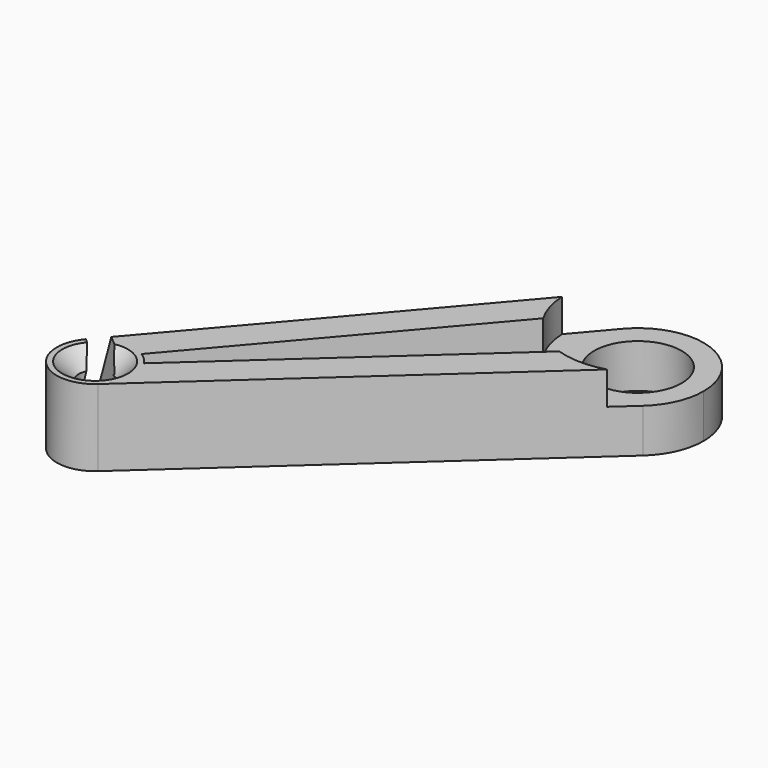
from build123d import *

# Parameters (mm, degrees)
F0_R     = 4
F0_R_2   = 1.5
F1_DEPTH = 7
F2_R     = 7.4
F3_DEPTH = 3
F4_SIZE  = 1.5
F6_DEPTH = 3


with BuildPart() as f1:
    # F0 (on Top) → F1 (new body)
    with BuildSketch(Plane.XY):
        with BuildLine():
            ThreePointArc((4.0311035144, -4.4441202117), (5.48573701, -2.4303681731), (6, 0))
            ThreePointArc((6, 0), (2.0737198646, 5.6302474122), (-4.5665619744, 3.8918519671))
            ThreePointArc((-4.5665619744, 3.8918519671), (-5.9006846613, 1.0871616841), (-5.6537236585, -2.0088326942))
            ThreePointArc((-5.6537236585, -2.0088326942), (-4.1765759878, -4.3076923077), (-1.8331692436, -5.7130981546))
            ThreePointArc((-1.8331692436, -5.7130981546), (1.2689779429, -5.864272758), (4.0311035144, -4.4441202117))
        make_face()
        Circle(F0_R, mode=Mode.SUBTRACT)
        with BuildLine():
            ThreePointArc((-5.6537236585, -2.0088326942), (-5.9006846613, 1.0871616841), (-4.5665619744, 3.8918519671))
            Line((-4.5665619744, 3.8918519671), (-29.8115717394, -25.7297530192))
            ThreePointArc((-29.8115717394, -25.7297530192), (-27.6751829567, -24.5399699331), (-25.2813289713, -25.0391732176))
            Line((-25.2813289713, -25.0391732176), (-5.6537236585, -2.0088326942))
        make_face()
        with BuildLine():
            Line((-24.7962668709, -30.5924034568), (4.0311035144, -4.4441202117))
            ThreePointArc((4.0311035144, -4.4441202117), (1.2689779429, -5.864272758), (-1.8331692436, -5.7130981546))
            Line((-1.8331692436, -5.7130981546), (-24.2460046276, -26.0429846518))
            ThreePointArc((-24.2460046276, -26.0429846518), (-23.8006490966, -26.9767912058), (-23.647743921, -28))
            ThreePointArc((-23.647743921, -28), (-23.9477306651, -29.4177147676), (-24.7962668709, -30.5924034568))
        make_face()
        with BuildLine():
            ThreePointArc((-25.2813289713, -25.0391732176), (-27.6751829567, -24.5399699331), (-29.8115717394, -25.7297530192))
            ThreePointArc((-29.8115717394, -25.7297530192), (-29.5840799139, -30.5128205128), (-24.7962668709, -30.5924034568))
            ThreePointArc((-24.7962668709, -30.5924034568), (-23.9477306651, -29.4177147676), (-23.647743921, -28))
            ThreePointArc((-23.647743921, -28), (-23.8006490966, -26.9767912058), (-24.2460046276, -26.0429846518))
            ThreePointArc((-24.2460046276, -26.0429846518), (-24.7114079281, -25.4871794872), (-25.2813289713, -25.0391732176))
        make_face()
        with Locations((-27.147743921, -28)):
            Circle(F0_R_2, mode=Mode.SUBTRACT)
    extrude(amount=F1_DEPTH)

    # F2 (on face) → F3 (cut)
    with BuildSketch(Plane.XY.offset(7)):
        with Locations((0, 0.9179179191)):
            Circle(F2_R)
    extrude(amount=-F3_DEPTH, mode=Mode.SUBTRACT)

    # F4
    f4_edges = [f1.edges().sort_by_distance(p)[0] for p in [
        (-28.647744, -28, 7),
    ]]
    chamfer(f4_edges, length=F4_SIZE)

    # F5 (on face) → F6 (cut)
    with BuildSketch(Plane(origin=(-4.5665619744, 3.8918519671, 0), x_dir=(-0.6486419945, -0.7610936624, 0), z_dir=(-0.7610936624, 0.6486419945, 0))):
        Polygon((40.5807819354, 0), (38.9197893108, 7), (38.9197893108, 0), align=None)
        Polygon((38.9197893108, 0), (38.9197893108, 7), (37.0698095831, 7), (38.7308022077, 0), align=None)
    extrude(amount=-F6_DEPTH, mode=Mode.SUBTRACT)


solid = f1.part
